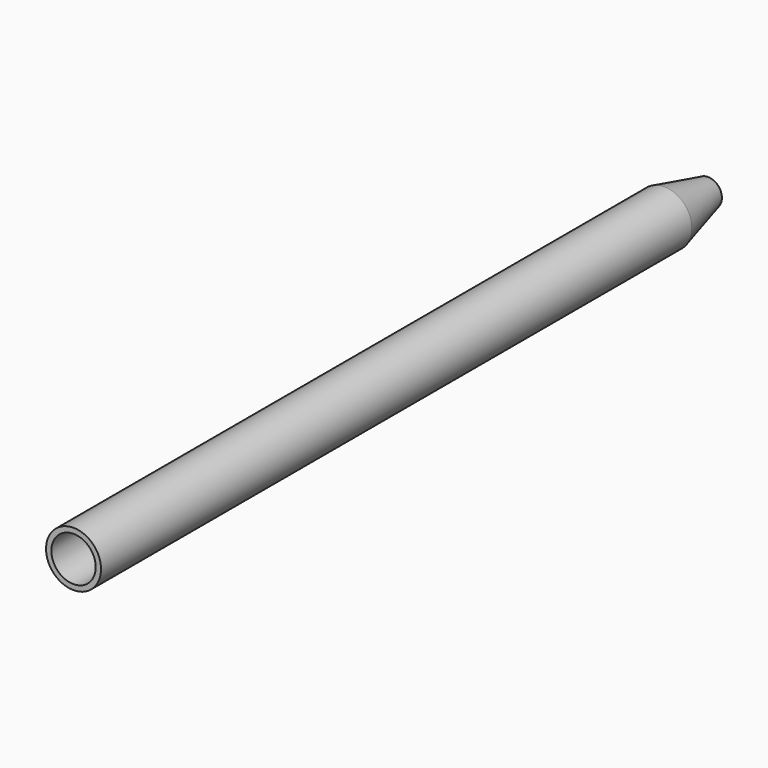
from build123d import *

# Parameters (mm, degrees)
F0_R     = 6.3836352682
F1_DEPTH = 171.45
F4_R     = 5.1492450533
F5_DEPTH = 171.45
F6_DEPTH = 12.7
F6_TAPER = 14
F8_DEPTH = 25.654


# Not quite as in the source:
# - the program builds the solid bodies; features that only make, move or delete a surface that nothing else refers to are left out


with BuildPart() as f1:
    # F0 (on Front) → F1 (new body)
    with BuildSketch(Plane.XZ):
        with Locations((-119.9116557837, -45.1905839145)):
            Circle(F0_R)
    extrude(amount=F1_DEPTH)

    # F4 (on Front) → F5 (cut)
    with BuildSketch(Plane.XZ):
        with Locations((-119.9116557837, -45.1905839145)):
            Circle(F4_R)
    extrude(amount=F5_DEPTH, mode=Mode.SUBTRACT)

    # F0 (on Front) → F6 (join)
    with BuildSketch(Plane.XZ):
        with Locations((-119.9116557837, -45.1905839145)):
            Circle(F0_R)
    extrude(amount=-F6_DEPTH, taper=F6_TAPER)

    # F8 (cut): a face of the model
    f8_faces = [f1.faces().sort_by_distance(p)[0] for p in [
        (-119.9116557837, 12.7, -45.1905839145),
    ]]
    extrude(f8_faces, amount=-F8_DEPTH, mode=Mode.SUBTRACT)


solid = f1.part
